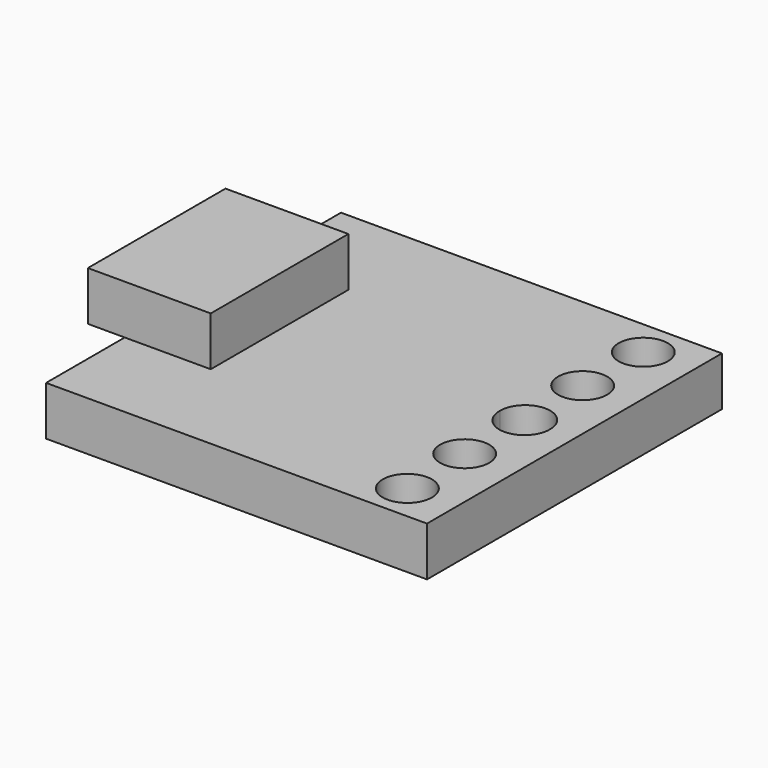
from build123d import *

# Parameters (mm, degrees)
F0_W     = 15.5
F0_H     = 15
F1_DEPTH = 2
F3_R     = 1
F3_R_2   = 1.0194429363
F4_DEPTH = 2
F5_W     = 5
F5_H     = 7
F6_DEPTH = 2


# Not quite as in the source:
# - a feature names something its author has since deleted; it is built from what else it names


with BuildPart() as f1:
    # F0 (on Top) → F1 (new body)
    with BuildSketch(Plane.XY):
        Rectangle(F0_W, F0_H)
    extrude(amount=F1_DEPTH)

    # F3 (on offset) → F4 (cut)
    with BuildSketch(Plane.XY.offset(2)):
        with Locations((5.75, 6)):
            Circle(F3_R)
        with Locations((5.6829168866, 3.0007501178)):
            Circle(F3_R)
        with Locations((5.7305570637, -0.0183169664)):
            Circle(F3_R_2)
        with Locations((5.7305570637, 0.0183169664)):
            Circle(F3_R_2)
        with Locations((5.6829168866, -3.0007501178)):
            Circle(F3_R)
        with Locations((5.75, -6)):
            Circle(F3_R)
    extrude(amount=-F4_DEPTH, mode=Mode.SUBTRACT)

    # F5 (on offset) → F6 (join)
    with BuildSketch(Plane.XY.offset(2)):
        with Locations((-6.75, 0)):
            Rectangle(F5_W, F5_H)
    extrude(amount=F6_DEPTH)


solid = f1.part
